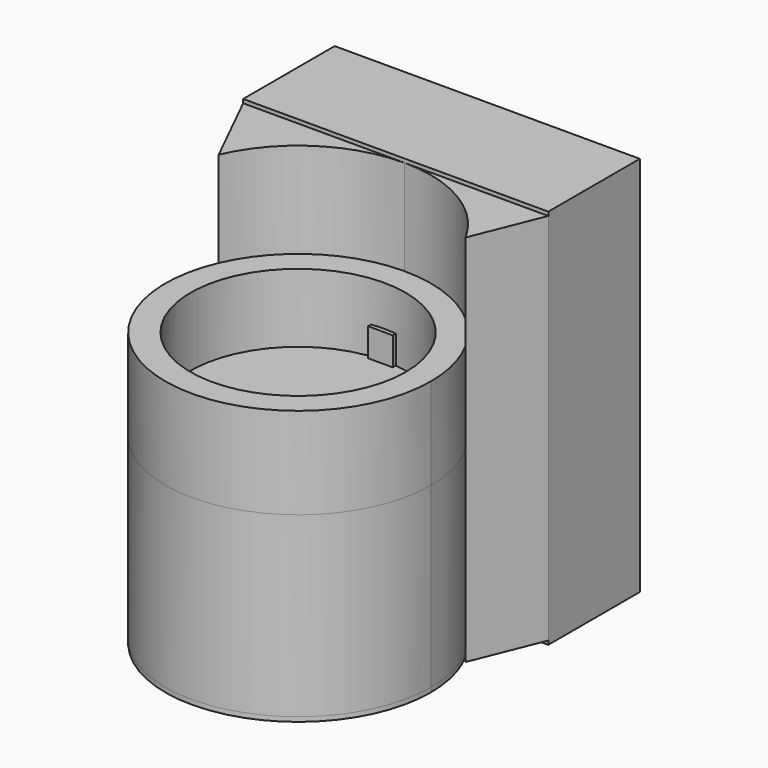
from build123d import *

# Parameters (mm, degrees)
F1_DEPTH = 63.5
F2_DEPTH = 62.23
F0_R     = 35.8003270569
F3_DEPTH = 60.706
F4_R     = 7.971733183
F6_DEPTH = 7.62
F7_DEPTH = 17.018
F8_DEPTH = 30.48
F9_DEPTH = 59.182


with BuildPart() as f1:
    # F0 (on Top) → F1 (new body, symmetric)
    with BuildSketch(Plane.XY):
        Polygon((-53.6557241526, 44.196), (0, 44.196), (47.9442758474, 44.196), (47.9442758474, 82.296), (-53.6557241526, 82.296), align=None)
    extrude(amount=F1_DEPTH, both=True)

    # F0 (on Top) → F2 (join, symmetric)
    with BuildSketch(Plane.XY):
        with BuildLine():
            Line((-53.6557241526, 44.196), (-40.5343907854, 17.6139030216))
            ThreePointArc((-40.5343907854, 17.6139030216), (-24.2365669811, 36.9577493494), (0, 44.196))
            Line((0, 44.196), (-53.6557241526, 44.196))
        make_face()
        with BuildLine():
            ThreePointArc((0, 44.196), (22.4909250619, 38.0452980782), (38.7217824253, 21.3051632664))
            Line((38.7217824253, 21.3051632664), (47.9442758474, 44.196))
            Line((47.9442758474, 44.196), (0, 44.196))
        make_face()
    extrude(amount=F2_DEPTH, both=True)

    # F0 (on Top) → F3 (join)
    with BuildSketch(Plane.XY):
        with BuildLine():
            ThreePointArc((-40.5343907854, 17.6139030216), (-8.9952343173, -43.2709160473), (44.196, 0))
            ThreePointArc((44.196, 0), (42.8055738898, 10.998602637), (38.7217824253, 21.3051632664))
            ThreePointArc((38.7217824253, 21.3051632664), (22.4909250619, 38.0452980782), (0, 44.196))
            ThreePointArc((0, 44.196), (-24.2365669811, 36.9577493494), (-40.5343907854, 17.6139030216))
        make_face()
        Circle(F0_R, mode=Mode.SUBTRACT)
    extrude(amount=-F3_DEPTH)

    # F4
    f4_edges = [f1.edges().sort_by_distance(p)[0] for p in [
        (-35.800327, 0, -60.706),
    ]]
    fillet(f4_edges, radius=F4_R)


with BuildPart() as f6:
    # F5 (on Top) → F6 (new body)
    with BuildSketch(Plane.XY):
        with BuildLine():
            Line((4.1009361986, 34.2692360282), (4.1009361986, 37.8786525935))
            ThreePointArc((4.1009361986, 37.8786525935), (0, 38.1), (-4.1009361986, 37.8786525935))
            Line((-4.1009361986, 37.8786525935), (-4.1009361986, 34.2692360282))
            Line((-4.1009361986, 34.2692360282), (4.1009361986, 34.2692360282))
        make_face()
        with BuildLine():
            ThreePointArc((-4.1009361986, 37.8786525935), (-25.4496004962, -28.3536211899), (38.1, 0))
            ThreePointArc((38.1, 0), (28.3536211899, 25.4496004962), (4.1009361986, 37.8786525935))
            Line((4.1009361986, 37.8786525935), (4.1009361986, 34.2692360282))
            Line((4.1009361986, 34.2692360282), (-4.1009361986, 34.2692360282))
            Line((-4.1009361986, 34.2692360282), (-4.1009361986, 37.8786525935))
        make_face()
    extrude(amount=F6_DEPTH)


with BuildPart() as f7:
    # F5 (on Top) → F7 (new body)
    with BuildSketch(Plane.XY):
        with BuildLine():
            Line((4.1009361986, 34.2692360282), (4.1009361986, 37.8786525935))
            ThreePointArc((4.1009361986, 37.8786525935), (0, 38.1), (-4.1009361986, 37.8786525935))
            Line((-4.1009361986, 37.8786525935), (-4.1009361986, 34.2692360282))
            Line((-4.1009361986, 34.2692360282), (4.1009361986, 34.2692360282))
        make_face()
    extrude(amount=F7_DEPTH)


with BuildPart() as f8:
    # F0 (on Top) → F8 (new body)
    with BuildSketch(Plane.XY):
        with BuildLine():
            ThreePointArc((-40.5343907854, 17.6139030216), (-8.9952343173, -43.2709160473), (44.196, 0))
            ThreePointArc((44.196, 0), (42.8055738898, 10.998602637), (38.7217824253, 21.3051632664))
            ThreePointArc((38.7217824253, 21.3051632664), (22.4909250619, 38.0452980782), (0, 44.196))
            ThreePointArc((0, 44.196), (-24.2365669811, 36.9577493494), (-40.5343907854, 17.6139030216))
        make_face()
        Circle(F0_R, mode=Mode.SUBTRACT)
    extrude(amount=F8_DEPTH)


with BuildPart() as f9:
    # F0 (on Top) → F9 (new body)
    with BuildSketch(Plane.XY):
        with BuildLine():
            ThreePointArc((-40.5343907854, 17.6139030216), (-8.9952343173, -43.2709160473), (44.196, 0))
            ThreePointArc((44.196, 0), (42.8055738898, 10.998602637), (38.7217824253, 21.3051632664))
            ThreePointArc((38.7217824253, 21.3051632664), (22.4909250619, 38.0452980782), (0, 44.196))
            ThreePointArc((0, 44.196), (-24.2365669811, 36.9577493494), (-40.5343907854, 17.6139030216))
        make_face()
        Circle(F0_R, mode=Mode.SUBTRACT)
    extrude(amount=-F9_DEPTH)


solid = Compound([f1.part, f6.part, f7.part, f8.part, f9.part])
